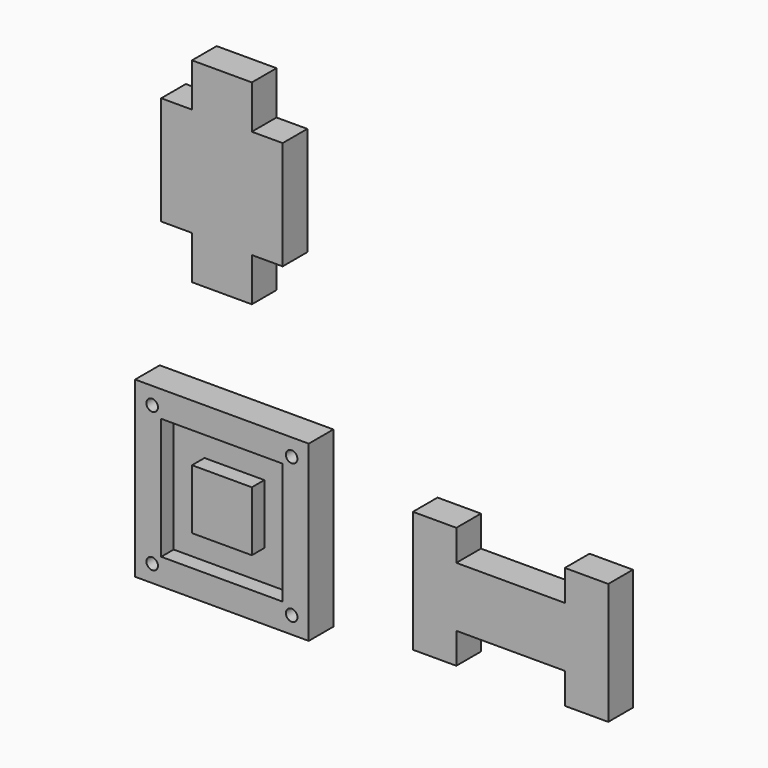
from build123d import *

# Parameters (mm, degrees)
F1_DEPTH = 18.034
F0_W     = 101.6
F0_H     = 101.6
F0_R     = 3.37439
F2_DEPTH = 8.89


# Not quite as in the source:
# - a feature names something its author has since deleted; it is built from what else it names


with BuildPart() as f1:
    # F0 (on Front) → F1 (new body)
    with BuildSketch(Plane.XZ):
        Polygon((-17.49933, 137.13333), (-17.49933, 111.73333), (17.49933, 111.73333), (17.49933, 137.13333), (35.53333, 137.13333), (35.53333, 200.63333), (17.49933, 200.63333), (17.49933, 226.03333), (-17.49933, 226.03333), (-17.49933, 200.63333), (-35.53333, 200.63333), (-35.53333, 137.13333), align=None)
    extrude(amount=F1_DEPTH)


with BuildPart() as f1b:
    # F0 (on Front) → F1, piece 2 (new body)
    with BuildSketch(Plane.XZ):
        Rectangle(F0_W, F0_H)
        with Locations((-40.80002, -40.80002)):
            Circle(F0_R, mode=Mode.SUBTRACT)
        with Locations((-40.80002, 40.80002)):
            Circle(F0_R, mode=Mode.SUBTRACT)
        with Locations((40.80002, -40.80002)):
            Circle(F0_R, mode=Mode.SUBTRACT)
        Polygon((35.53333, 35.53333), (35.53333, 17.49933), (35.53333, -17.49933), (35.53333, -35.53333), (-35.53333, -35.53333), (-35.53333, -17.49933), (-35.53333, 17.49933), (-35.53333, 35.53333), align=None, mode=Mode.SUBTRACT)
        with Locations((40.80002, 40.80002)):
            Circle(F0_R, mode=Mode.SUBTRACT)
    extrude(amount=F1_DEPTH)



with BuildPart() as f1c:
    # F0 (on Front) → F1, piece 3 (new body)
    with BuildSketch(Plane.XZ):
        with BuildLine():
            ThreePointArc((5.04e-08, 17.49933), (12.373894927, 12.3738948914), (17.49933, 0))
            Line((17.49933, 0), (17.49933, 17.49933))
            Line((17.49933, 17.49933), (5.04e-08, 17.49933))
        make_face()
        with BuildLine():
            ThreePointArc((-17.49933, 1.35e-08), (-12.3738948866, 12.3738949318), (5.04e-08, 17.49933))
            Line((5.04e-08, 17.49933), (-17.49933, 17.49933))
            Line((-17.49933, 17.49933), (-17.49933, 1.35e-08))
        make_face()
        with BuildLine():
            ThreePointArc((1.06e-08, -17.49933), (12.373894913, -12.3738949055), (17.49933, 0))
            ThreePointArc((17.49933, 0), (12.373894927, 12.3738948914), (5.04e-08, 17.49933))
            ThreePointArc((5.04e-08, 17.49933), (-12.3738948866, 12.3738949318), (-17.49933, 1.35e-08))
            ThreePointArc((-17.49933, 1.35e-08), (-12.3738949102, -12.3738949082), (1.06e-08, -17.49933))
        make_face()
        with BuildLine():
            Line((-17.49933, -17.49933), (1.06e-08, -17.49933))
            ThreePointArc((1.06e-08, -17.49933), (-12.3738949102, -12.3738949082), (-17.49933, 1.35e-08))
            Line((-17.49933, 1.35e-08), (-17.49933, -17.49933))
        make_face()
        with BuildLine():
            Line((17.49933, -17.49933), (17.49933, 0))
            ThreePointArc((17.49933, 0), (12.373894913, -12.3738949055), (1.06e-08, -17.49933))
            Line((1.06e-08, -17.49933), (17.49933, -17.49933))
        make_face()
    extrude(amount=F1_DEPTH)


with BuildPart() as f1d:
    # F0 (on Front) → F1, piece 4 (new body)
    with BuildSketch(Plane.XZ):
        Polygon((137.13333, 35.53333), (111.73333, 35.53333), (111.73333, -35.53333), (137.13333, -35.53333), (137.13333, -17.49933), (200.63333, -17.49933), (200.63333, -35.53333), (226.03333, -35.53333), (226.03333, 35.53333), (200.63333, 35.53333), (200.63333, 17.49933), (137.13333, 17.49933), align=None)
    extrude(amount=F1_DEPTH)


with BuildPart() as f1b_1:
    add(f1b.part)

    add(f1c.part)  # F2 merges F1c
    # F0 (on Front) → F2 (join)
    with BuildSketch(Plane.XZ):
        Polygon((-17.49933, 17.49933), (5.04e-08, 17.49933), (17.49933, 17.49933), (35.53333, 17.49933), (35.53333, 35.53333), (-35.53333, 35.53333), (-35.53333, 17.49933), align=None)
        Polygon((-17.49933, -17.49933), (-17.49933, 1.35e-08), (-17.49933, 17.49933), (-35.53333, 17.49933), (-35.53333, -17.49933), align=None)
        Polygon((17.49933, -17.49933), (1.06e-08, -17.49933), (-17.49933, -17.49933), (-35.53333, -17.49933), (-35.53333, -35.53333), (35.53333, -35.53333), (35.53333, -17.49933), align=None)
        Polygon((17.49933, 17.49933), (17.49933, 0), (17.49933, -17.49933), (35.53333, -17.49933), (35.53333, 17.49933), align=None)
    extrude(amount=F2_DEPTH)


solid = Compound([f1.part, f1d.part, f1b_1.part])
